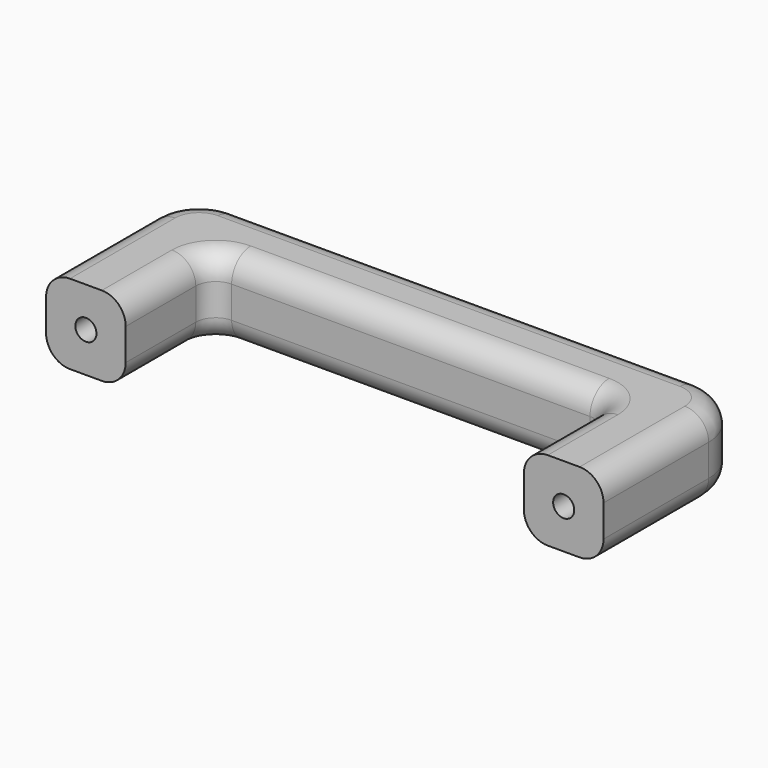
from build123d import *

# Parameters (mm, degrees)
F0_W          = 140
F0_H          = 45
F1_DEPTH      = 20
F2_W          = 100
F2_H          = 27
F3_DEPTH      = 25
F4_R          = 2.65
F5_DEPTH      = 45.001
F6_R          = 4.5
F7_DEPTH      = 25
F8_T1_DEPTH   = 80
F9_R          = 5
F10_T1_DEPTH  = 116
F10_T3_DEPTH  = 90
F10_T5_DEPTH  = 37
F10_T7_DEPTH  = 48
F10_T10_ANGLE = 90
F10_T12_ANGLE = 90
F10_T14_ANGLE = 89.9999999987
F10_T16_ANGLE = 89.9999999987
F10_T18_ANGLE = 90
F10_T20_ANGLE = 90
F10_T22_ANGLE = 89.9999999987
F10_T24_ANGLE = 89.9999999987


# Not quite as in the source:
# - a fillet or chamfer that OpenCascade refuses, or shapes differently, is made with other operations: its cross-section is extruded or revolved along the edge and cut away or added


with BuildPart() as f1:
    # F0 (on Top) → F1 (new body)
    with BuildSketch(Plane.XY):
        Rectangle(F0_W, F0_H)
    extrude(amount=F1_DEPTH)

    # F2 (on face) → F3 (cut)
    with BuildSketch(Plane.XY.offset(20)):
        with Locations((0, -9)):
            Rectangle(F2_W, F2_H)
    extrude(amount=-F3_DEPTH, mode=Mode.SUBTRACT)

    # F4 (on face) → F5 (cut, through all)
    with BuildSketch(Plane(origin=(0, 22.5, 0), x_dir=(-1, 0, 0), z_dir=(0, 1, 0))):
        with Locations((60, 10)):
            Circle(F4_R)
        with Locations((-60, 10)):
            Circle(F4_R)
    extrude(amount=-F5_DEPTH, mode=Mode.SUBTRACT)

    # F6 (on face) → F7 (cut)
    with BuildSketch(Plane(origin=(0, 22.5, 0), x_dir=(-1, 0, 0), z_dir=(0, 1, 0))):
        with Locations((60, 10)):
            Circle(F6_R)
        with Locations((-60, 10)):
            Circle(F6_R)
    extrude(amount=-F7_DEPTH, mode=Mode.SUBTRACT)

    # F8: fillet of radius 12 on 2 edges, made by hand

    # F8_s2 → F8_t1 (cut)
    with BuildSketch(Plane.XY.offset(-30)):
        with BuildLine():
            ThreePointArc((-58, 22.5), (-66.4852813742, 18.9852813742), (-70, 10.5))
            Line((-70, 10.5), (-70, 22.5))
            Line((-70, 22.5), (-58, 22.5))
        make_face()
        with BuildLine():
            ThreePointArc((58, 22.5), (66.4852813742, 18.9852813742), (70, 10.5))
            Line((70, 10.5), (70, 22.5))
            Line((70, 22.5), (58, 22.5))
        make_face()
    extrude(amount=F8_T1_DEPTH, mode=Mode.SUBTRACT)

    # F9
    f9_edges = [f1.edges().sort_by_distance(p)[0] for p in [
        (-50, 4.5, 10),
        (50, 4.5, 10),
    ]]
    fillet(f9_edges, radius=F9_R)

    # F10: fillet of radius 6 on 20 edges, made by hand

    # F10_s2 → F10_t1 (cut)
    with BuildSketch(Plane.YZ.offset(-58)):
        with BuildLine():
            ThreePointArc((22.5, 14), (20.7426406871, 18.2426406871), (16.5, 20))
            Line((16.5, 20), (22.5, 20))
            Line((22.5, 20), (22.5, 14))
        make_face()
        with BuildLine():
            ThreePointArc((16.5, 0), (20.7426406871, 1.7573593129), (22.5, 6))
            Line((22.5, 6), (22.5, 0))
            Line((22.5, 0), (16.5, 0))
        make_face()
    extrude(amount=F10_T1_DEPTH, mode=Mode.SUBTRACT)

    # F10_s4 → F10_t3 (cut)
    with BuildSketch(Plane.YZ.offset(-45)):
        with BuildLine():
            ThreePointArc((4.5, 14), (6.2573593129, 18.2426406871), (10.5, 20))
            Line((10.5, 20), (4.5, 20))
            Line((4.5, 20), (4.5, 14))
        make_face()
        with BuildLine():
            ThreePointArc((10.5, 0), (6.2573593129, 1.7573593129), (4.5, 6))
            Line((4.5, 6), (4.5, 0))
            Line((4.5, 0), (10.5, 0))
        make_face()
    extrude(amount=F10_T3_DEPTH, mode=Mode.SUBTRACT)

    # F10_s6 → F10_t5 (cut)
    with BuildSketch(Plane.XZ.offset(0.5)):
        with BuildLine():
            ThreePointArc((56, 0), (51.7573593129, 1.7573593129), (50, 6))
            Line((50, 6), (50, 0))
            Line((50, 0), (56, 0))
        make_face()
        with BuildLine():
            ThreePointArc((-56, 0), (-51.7573593129, 1.7573593129), (-50, 6))
            Line((-50, 6), (-50, 0))
            Line((-50, 0), (-56, 0))
        make_face()
        with BuildLine():
            ThreePointArc((50, 14), (51.7573593129, 18.2426406871), (56, 20))
            Line((56, 20), (50, 20))
            Line((50, 20), (50, 14))
        make_face()
        with BuildLine():
            ThreePointArc((-50, 14), (-51.7573593129, 18.2426406871), (-56, 20))
            Line((-56, 20), (-50, 20))
            Line((-50, 20), (-50, 14))
        make_face()
    extrude(amount=F10_T5_DEPTH, mode=Mode.SUBTRACT)

    # F10_s8 → F10_t7 (cut)
    with BuildSketch(Plane.XZ.offset(-10.5)):
        with BuildLine():
            ThreePointArc((64, 0), (68.2426406871, 1.7573593129), (70, 6))
            Line((70, 6), (70, 0))
            Line((70, 0), (64, 0))
        make_face()
        with BuildLine():
            ThreePointArc((-64, 0), (-68.2426406871, 1.7573593129), (-70, 6))
            Line((-70, 6), (-70, 0))
            Line((-70, 0), (-64, 0))
        make_face()
        with BuildLine():
            ThreePointArc((70, 14), (68.2426406871, 18.2426406871), (64, 20))
            Line((64, 20), (70, 20))
            Line((70, 20), (70, 14))
        make_face()
        with BuildLine():
            ThreePointArc((-70, 14), (-68.2426406871, 18.2426406871), (-64, 20))
            Line((-64, 20), (-70, 20))
            Line((-70, 20), (-70, 14))
        make_face()
    extrude(amount=F10_T7_DEPTH, mode=Mode.SUBTRACT)

    # F10_s9 → F10_t10 (revolve, cut)
    with BuildSketch(Plane.XZ.offset(0.5)):
        with BuildLine():
            ThreePointArc((56, 0), (51.7573593129, 1.7573593129), (50, 6))
            Line((50, 6), (50, 0))
            Line((50, 0), (56, 0))
        make_face()
    revolve(axis=Axis((45, -0.5, 0), (0, 0, 1)), revolution_arc=F10_T10_ANGLE, mode=Mode.SUBTRACT)

    # F10_s11 → F10_t12 (revolve, cut)
    with BuildSketch(Plane.YZ.offset(-45)):
        with BuildLine():
            ThreePointArc((10.5, 0), (6.2573593129, 1.7573593129), (4.5, 6))
            Line((4.5, 6), (4.5, 0))
            Line((4.5, 0), (10.5, 0))
        make_face()
    revolve(axis=Axis((-45, -0.5, 0), (0, 0, 1)), revolution_arc=F10_T12_ANGLE, mode=Mode.SUBTRACT)

    # F10_s13 → F10_t14 (revolve, cut)
    with BuildSketch(Plane.YZ.offset(57.9999999999)):
        with BuildLine():
            ThreePointArc((16.5, 0), (20.7426406871, 1.7573593129), (22.5, 6))
            Line((22.5, 6), (22.5, 0))
            Line((22.5, 0), (16.5, 0))
        make_face()
    revolve(axis=Axis((57.9999999999, 10.4999999999, 0), (0, 0, -1)), revolution_arc=F10_T14_ANGLE, mode=Mode.SUBTRACT)

    # F10_s15 → F10_t16 (revolve, cut)
    with BuildSketch(Plane.XZ.offset(-10.4999999999)):
        with BuildLine():
            ThreePointArc((-64, 0), (-68.2426406871, 1.7573593129), (-70, 6))
            Line((-70, 6), (-70, 0))
            Line((-70, 0), (-64, 0))
        make_face()
    revolve(axis=Axis((-57.9999999999, 10.4999999999, 0), (0, 0, -1)), revolution_arc=F10_T16_ANGLE, mode=Mode.SUBTRACT)

    # F10_s17 → F10_t18 (revolve, cut)
    with BuildSketch(Plane.XZ.offset(0.5)):
        with BuildLine():
            ThreePointArc((50, 14), (51.7573593129, 18.2426406871), (56, 20))
            Line((56, 20), (50, 20))
            Line((50, 20), (50, 14))
        make_face()
    revolve(axis=Axis((45, -0.5, 20), (0, 0, 1)), revolution_arc=F10_T18_ANGLE, mode=Mode.SUBTRACT)

    # F10_s19 → F10_t20 (revolve, cut)
    with BuildSketch(Plane.YZ.offset(-45)):
        with BuildLine():
            ThreePointArc((4.5, 14), (6.2573593129, 18.2426406871), (10.5, 20))
            Line((10.5, 20), (4.5, 20))
            Line((4.5, 20), (4.5, 14))
        make_face()
    revolve(axis=Axis((-45, -0.5, 20), (0, 0, 1)), revolution_arc=F10_T20_ANGLE, mode=Mode.SUBTRACT)

    # F10_s21 → F10_t22 (revolve, cut)
    with BuildSketch(Plane.YZ.offset(57.9999999999)):
        with BuildLine():
            ThreePointArc((22.5, 14), (20.7426406871, 18.2426406871), (16.5, 20))
            Line((16.5, 20), (22.5, 20))
            Line((22.5, 20), (22.5, 14))
        make_face()
    revolve(axis=Axis((57.9999999999, 10.4999999999, 20), (0, 0, -1)), revolution_arc=F10_T22_ANGLE, mode=Mode.SUBTRACT)

    # F10_s23 → F10_t24 (revolve, cut)
    with BuildSketch(Plane.XZ.offset(-10.4999999999)):
        with BuildLine():
            ThreePointArc((-70, 14), (-68.2426406871, 18.2426406871), (-64, 20))
            Line((-64, 20), (-70, 20))
            Line((-70, 20), (-70, 14))
        make_face()
    revolve(axis=Axis((-57.9999999999, 10.4999999999, 20), (0, 0, -1)), revolution_arc=F10_T24_ANGLE, mode=Mode.SUBTRACT)


solid = f1.part
